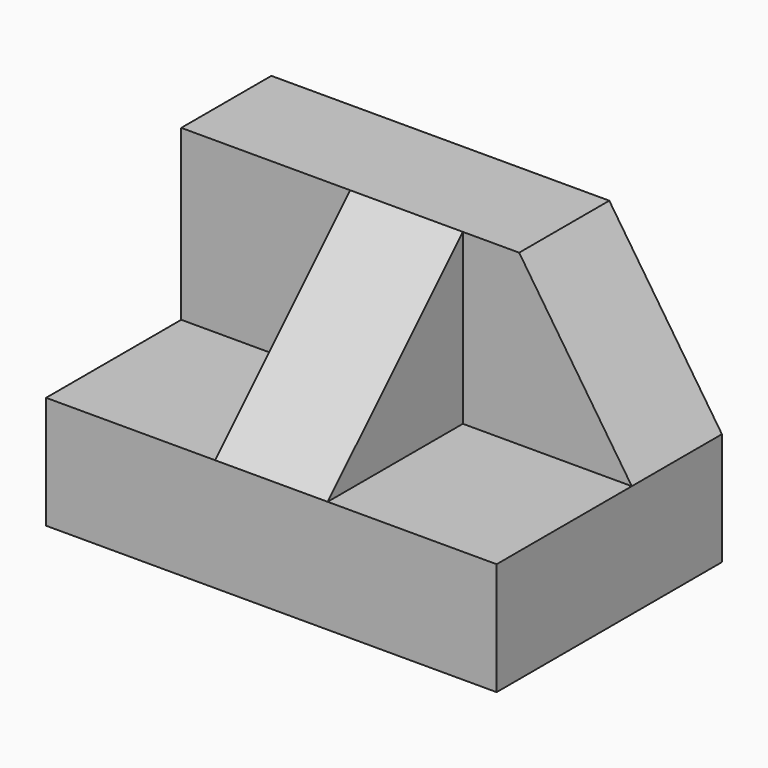
from build123d import *

# Parameters (mm, degrees)
F1_DEPTH = 50.8
F3_DEPTH = 25.4
F5_DEPTH = 31.75
F6_W     = 12.7
F6_H     = 26.9407683632
F7_DEPTH = 19.05
F8_W     = 19.05
F8_H     = 26.9407683632
F9_DEPTH = 19.05


with BuildPart() as f1:
    # F0 (on Right) → F1 (new body)
    with BuildSketch(Plane.YZ):
        Polygon((0, 12.7), (0, 0), (31.75, 0), (31.75, 31.75), (19.05, 31.75), (19.05, 12.7), align=None)
    extrude(amount=F1_DEPTH)

    # F2 (on face) → F3 (cut)
    with BuildSketch(Plane.XZ.offset(-19.05)):
        Polygon((38.1, 31.75), (50.8, 12.7), (50.8, 31.75), align=None)
    extrude(amount=-F3_DEPTH, mode=Mode.SUBTRACT)

    # F6 (on face) → F7 (cut)
    with BuildSketch(Plane(origin=(0, -6.35, 6.35), x_dir=(1, 0, 0), z_dir=(0, -0.7071067812, 0.7071067812))):
        with Locations((25.4, 22.4506403027)):
            Rectangle(F6_W, F6_H)
    extrude(amount=F7_DEPTH, mode=Mode.SUBTRACT)


with BuildPart() as f5:
    # F4 (on face) → F5 (new body)
    with BuildSketch(Plane(origin=(0, 0, 0), x_dir=(0, -1, 0), z_dir=(-1, 0, 0))):
        Polygon((0, 12.7), (-19.05, 31.75), (-19.05, 12.7), align=None)
    extrude(amount=-F5_DEPTH)

    # F8 (on face) → F9 (cut)
    with BuildSketch(Plane(origin=(0, -6.35, 6.35), x_dir=(1, 0, 0), z_dir=(0, -0.7071067812, 0.7071067812))):
        with Locations((9.525, 22.4506403027)):
            Rectangle(F8_W, F8_H)
    extrude(amount=-F9_DEPTH, mode=Mode.SUBTRACT)


solid = Compound([f1.part, f5.part])
